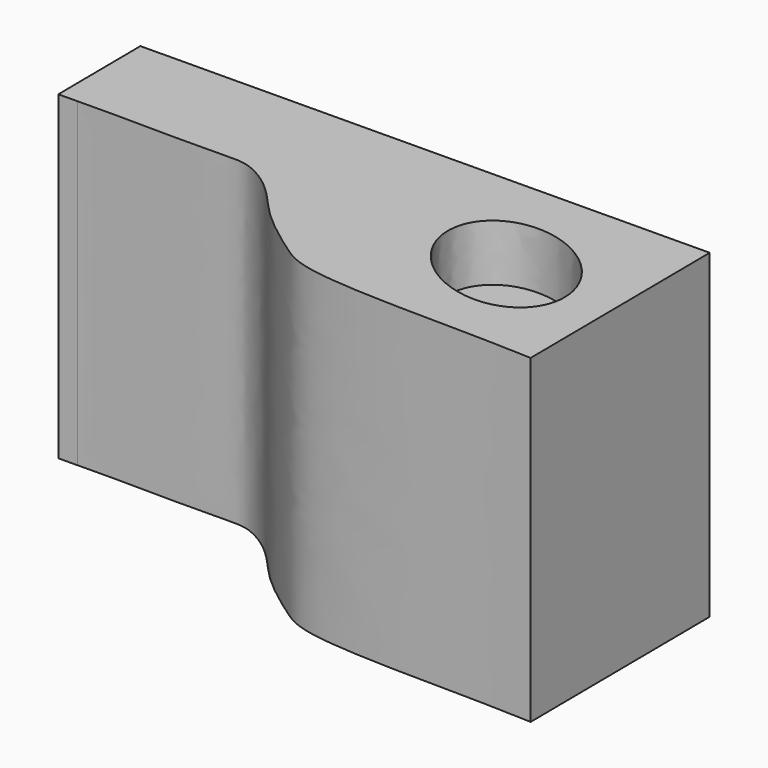
from build123d import *

# Parameters (mm, degrees)
F1_DEPTH = 863.6
F3_DEPTH = 152.4


with BuildPart() as f1:
    # F0 (on Top) → F1 (new body)
    with BuildSketch(Plane.XY):
        with BuildLine():
            Line((5.1712791552, -609.5780654452), (0, 0))
            Line((0, 0), (-1523.945163613, -12.9281978881))
            Line((-1523.945163613, -12.9281978881), (-1521.5749940002, -292.3181445505))
            Line((-1521.5749940002, -292.3181445505), (-1470.267745312, -291.8828859336))
            add(Edge.make_bspline(
                [(-1470.267745312, -291.8828859336), (-1417.5702780767, -289.2463226551), (-1095.5111979406, -295.9816219873), (-1009.8644785837, -285.5675139686), (-908.1150816583, -351.6452825618), (-837.6932292983, -445.1648141807), (-712.3005781961, -536.8126968936), (-628.5880833926, -594.1331007539), (-339.4123112672, -603.9797790496), (-131.2186034217, -604.0444126029), (-49.0435831404, -607.9862117262), (5.1712791552, -609.5780654452)],
                knots=[0, 0, 0, 0, 0.1645442885, 0.2521608346, 0.3403282662, 0.4361793801, 0.5413406025, 0.6281413427, 0.7734172402, 0.8991700782, 1, 1, 1, 1], degree=3))
        make_face()
    extrude(amount=F1_DEPTH)

    # F2 (on face) → F3 (cut)
    with BuildSketch(Plane.XY.offset(863.6)):
        with BuildLine():
            add(Edge.make_bspline(
                [(-129.1464435727, -413.8713023162), (9.1967369441, -189.0637303697), (-319.5602776727, -141.722571319), (-648.3172922894, -94.3814122683), (-457.9034581895, -366.5301432655), (-267.4896240896, -638.6788742627), (-129.1464435727, -413.8713023162)],
                knots=[0, 0, 0, 2.0943951024, 2.0943951024, 4.1887902048, 4.1887902048, 6.2831853072, 6.2831853072, 6.2831853072], degree=2, weights=[1, 0.5, 1, 0.5, 1, 0.5, 1]))
        make_face()
    extrude(amount=-F3_DEPTH, mode=Mode.SUBTRACT)


solid = f1.part
